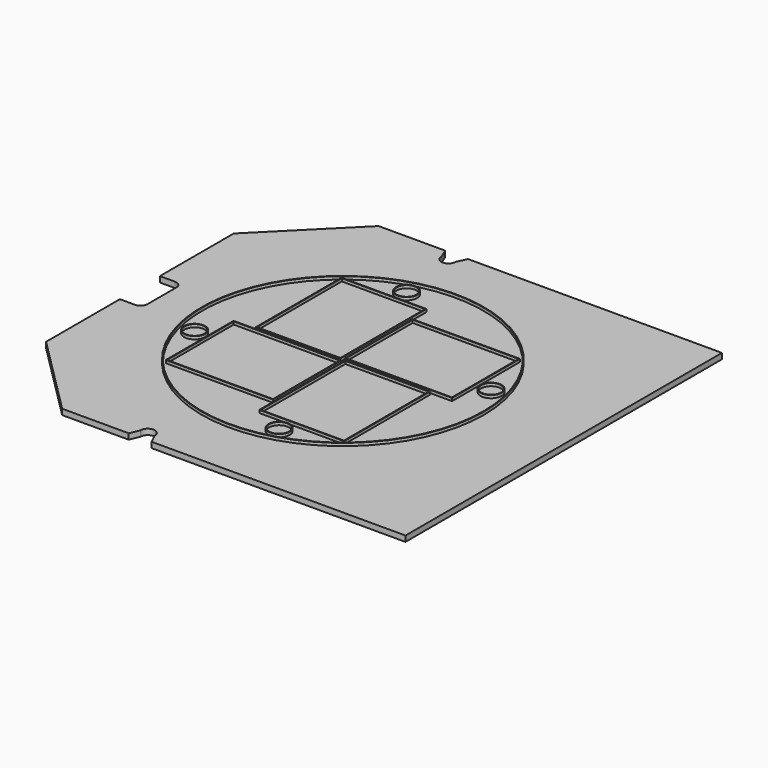
from build123d import *

# Parameters (mm, degrees)
F0_W     = 150
F0_H     = 140
F1_DEPTH = 2
F2_R     = 2.5
F3_DEPTH = 5
F4_R     = 50
F4_R_2   = 49.75
F5_DEPTH = 1
F6_DEPTH = 1
F4_W     = 38
F4_H     = 30
F4_W_2   = 37.5
F4_H_2   = 29.5
F4_R_3   = 3.75
F4_R_4   = 3.5
F4_W_3   = 30
F4_H_3   = 38
F4_W_4   = 29.5
F4_H_4   = 37.5


# Not quite as in the source:
# - a feature names something its author has since deleted; it is built from what else it names


with BuildPart() as f1:
    # F0 (on Top) → F1 (new body)
    with BuildSketch(Plane.XY):
        Rectangle(F0_W, F0_H)
    extrude(amount=F1_DEPTH)

    # F2 (on face) → F3 (cut)
    with BuildSketch(Plane.XY.offset(2)):
        Polygon((-75, 70), (-75, 41.5), (-46.5, 70), align=None)
        with Locations((-64, 57.6)):
            Circle(F2_R, mode=Mode.SUBTRACT)
        Polygon((-46.5, -70), (-75, -41.5), (-75, -70), align=None)
        with Locations((-64, -57.6)):
            Circle(F2_R, mode=Mode.SUBTRACT)
        with BuildLine():
            Line((-67.1845650673, -6.35), (-67.1845650673, 6.35))
            ThreePointArc((-67.1845650673, 6.35), (-67.9167981143, 8.117766953), (-69.6845650673, 8.85))
            Line((-69.6845650673, 8.85), (-75, 8.85))
            Line((-75, 8.85), (-75, -8.85))
            Line((-75, -8.85), (-69.6845650673, -8.85))
            ThreePointArc((-69.6845650673, -8.85), (-67.9167981143, -8.117766953), (-67.1845650673, -6.35))
        make_face()
        with BuildLine():
            Line((-21.499911428, -66.5210440509), (-22.940942165, -70))
            Line((-22.940942165, -70), (-14.8778247705, -70))
            Line((-14.8778247705, -70), (-16.500088572, -66.5210440509))
            ThreePointArc((-16.500088572, -66.5210440509), (-19, -64), (-21.499911428, -66.5210440509))
        make_face()
        with BuildLine():
            Line((-14.8778247705, 70), (-22.940942165, 70))
            Line((-22.940942165, 70), (-21.499911428, 66.5210440509))
            ThreePointArc((-21.499911428, 66.5210440509), (-19, 64), (-16.500088572, 66.5210440509))
            Line((-16.500088572, 66.5210440509), (-14.8778247705, 70))
        make_face()
        with Locations((-64, 57.6)):
            Circle(F2_R)
        with Locations((-64, -57.6)):
            Circle(F2_R)
    extrude(amount=-F3_DEPTH, mode=Mode.SUBTRACT)


with BuildPart() as f5:
    # F4 (on face) → F5 (new body)
    with BuildSketch(Plane.XY.offset(2)):
        with Locations((-3.1632825379, 0)):
            Circle(F4_R)
        with Locations((-3.1632825379, 0)):
            Circle(F4_R_2, mode=Mode.SUBTRACT)
    extrude(amount=F5_DEPTH)


with BuildPart() as f6:
    # F4 (on face) → F6 (new body)
    with BuildSketch(Plane.XY.offset(2)):
        with Locations((-3.1632825379, 0)):
            Circle(F4_R)
        with Locations((-3.1632825379, 0)):
            Circle(F4_R_2, mode=Mode.SUBTRACT)
    extrude(amount=F6_DEPTH)


with BuildPart() as f6b:
    # F4 (on face) → F6, piece 2 (new body)
    with BuildSketch(Plane.XY.offset(2)):
        with Locations((-22.1632825379, -15.8367174621)):
            Rectangle(F4_W, F4_H)
        with Locations((-22.1632825379, -15.8367174621)):
            Rectangle(F4_W_2, F4_H_2, mode=Mode.SUBTRACT)
    extrude(amount=F6_DEPTH)


with BuildPart() as f6c:
    # F4 (on face) → F6, piece 3 (new body)
    with BuildSketch(Plane.XY.offset(2)):
        with Locations((-46.1632825379, -11.8367174621)):
            Circle(F4_R_3)
        with Locations((-46.1632825379, -11.8367174621)):
            Circle(F4_R_4, mode=Mode.SUBTRACT)
    extrude(amount=F6_DEPTH)


with BuildPart() as f6d:
    # F4 (on face) → F6, piece 4 (new body)
    with BuildSketch(Plane.XY.offset(2)):
        with Locations((-19, 19)):
            Rectangle(F4_W_3, F4_H_3)
        with Locations((-19, 19)):
            Rectangle(F4_W_4, F4_H_4, mode=Mode.SUBTRACT)
    extrude(amount=F6_DEPTH)


with BuildPart() as f6e:
    # F4 (on face) → F6, piece 5 (new body)
    with BuildSketch(Plane.XY.offset(2)):
        with Locations((15.8367174621, 15.8367174621)):
            Rectangle(F4_W, F4_H)
        with Locations((15.8367174621, 15.8367174621)):
            Rectangle(F4_W_2, F4_H_2, mode=Mode.SUBTRACT)
    extrude(amount=F6_DEPTH)


with BuildPart() as f6f:
    # F4 (on face) → F6, piece 6 (new body)
    with BuildSketch(Plane.XY.offset(2)):
        with Locations((12.6734349243, -19)):
            Rectangle(F4_W_3, F4_H_3)
        with Locations((12.6734349243, -19)):
            Rectangle(F4_W_4, F4_H_4, mode=Mode.SUBTRACT)
    extrude(amount=F6_DEPTH)


with BuildPart() as f6g:
    # F4 (on face) → F6, piece 7 (new body)
    with BuildSketch(Plane.XY.offset(2)):
        with Locations((39.8367174621, 11.8367174621)):
            Circle(F4_R_3)
        with Locations((39.8367174621, 11.8367174621)):
            Circle(F4_R_4, mode=Mode.SUBTRACT)
    extrude(amount=F6_DEPTH)


with BuildPart() as f6h:
    # F4 (on face) → F6, piece 8 (new body)
    with BuildSketch(Plane.XY.offset(2)):
        with Locations((8.6734349243, -43)):
            Circle(F4_R_3)
        with Locations((8.6734349243, -43)):
            Circle(F4_R_4, mode=Mode.SUBTRACT)
    extrude(amount=F6_DEPTH)


with BuildPart() as f6i:
    # F4 (on face) → F6, piece 9 (new body)
    with BuildSketch(Plane.XY.offset(2)):
        with Locations((-15, 43)):
            Circle(F4_R_3)
        with Locations((-15, 43)):
            Circle(F4_R_4, mode=Mode.SUBTRACT)
    extrude(amount=F6_DEPTH)


solid = Compound([f1.part, f5.part, f6.part, f6b.part, f6c.part, f6d.part, f6e.part, f6f.part, f6g.part, f6h.part, f6i.part])
